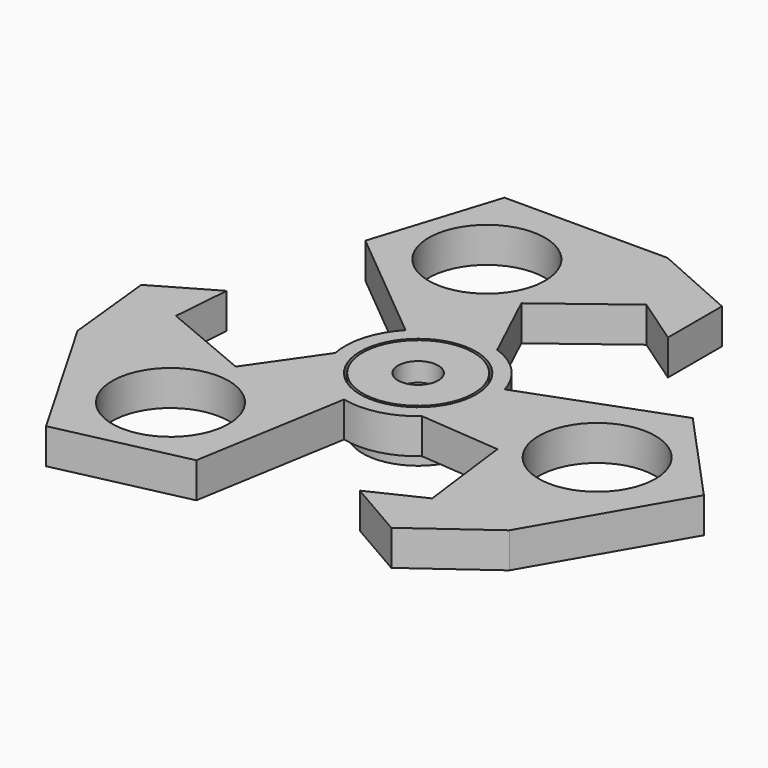
from build123d import *

# Parameters (mm, degrees)
F0_R            = 11
F0_R_2          = 4
F1_DEPTH        = 7
F3_R            = 14.5
F3_R_2          = 11.5
F4_DEPTH        = 7
F2_R            = 11.5528949888
F5_DEPTH        = 7
F5_COPIES_COUNT = 3
F6_R            = 3.4998709427
F7_DEPTH        = 3.5
F8_DEPTH        = 1


# Not quite as in the source:
# - a pattern or mirror of a feature is missing from the dataset's text; its kind, count and spacing are read off the source's solid


with BuildPart() as f1:
    # F0 (on Top) → F1 (new body)
    with BuildSketch(Plane.XY):
        Circle(F0_R)
        Circle(F0_R_2, mode=Mode.SUBTRACT)
    extrude(amount=F1_DEPTH)


with BuildPart() as f4:
    # F3 (on Top) → F4 (new body)
    with BuildSketch(Plane.XY):
        Circle(F3_R)
        Circle(F3_R_2, mode=Mode.SUBTRACT)
    extrude(amount=F4_DEPTH)

    # F2 (on Top) → F5 (join)
    with BuildSketch(Plane.XY):
        with BuildLine():
            ThreePointArc((-8.1796808061, 8.0834907009), (-0.9163388311, 11.4634341777), (6.7916970403, 9.2802398305))
            Line((6.7916970403, 9.2802398305), (-2.1384290885, 28.2644629478))
            Line((-2.1384290885, 28.2644629478), (13.2954539731, 39.9793423712))
            Line((13.2954539731, 39.9793423712), (22.7789282799, 33.4710739553))
            Line((22.7789282799, 33.4710739553), (22.7789282799, 46.8595065176))
            Line((22.7789282799, 46.8595065176), (6.0433889739, 54.2975254357))
            Line((6.0433889739, 54.2975254357), (-26.3119842857, 54.2975254357))
            Line((-26.3119842857, 54.2975254357), (-34.1219007969, 29.566116631))
            Line((-34.1219007969, 29.566116631), (-8.1796808061, 8.0834907009))
        make_face()
        with Locations((-15.5268600211, 36.4462845027)):
            Circle(F2_R, mode=Mode.SUBTRACT)
    f5 = extrude(amount=F5_DEPTH)

    # F5_copies: F5 ×3 about axis
    f5_copies_axis = Axis((0, 0, 0), (0, 0, 1))
    for i in range(1, F5_COPIES_COUNT):
        add(f5.rotate(f5_copies_axis, i * 360 / F5_COPIES_COUNT))


with BuildPart() as f7:
    # F6 (on Top) → F7 (new body)
    with BuildSketch(Plane.XY):
        Circle(F6_R)
    extrude(amount=F7_DEPTH)

    # F8 (add): a face of the model
    f8_faces = [f7.faces().sort_by_distance(p)[0] for p in [
        (0, 0, 0),
    ]]
    extrude(f8_faces, amount=F8_DEPTH)

    # F9 (on Right) → F10 (revolve)
    with BuildSketch(Plane.YZ):
        Polygon((10.9668523421, -3.5042045906), (11, -0.5043877241), (0, -0.5043877241), (0, -1.8302736931), (7.2377983444, -1.8302736931), (7.8344469729, -1.9960094697), (8.3648014024, -2.2280394454), (8.9614500308, -2.5097902099), (9.9558646908, -2.9904239901), align=None)
    revolve(axis=Axis((0, 0, -1.1673307086), (0, 0, -1)))


solid = Compound([f1.part, f4.part, f7.part])
